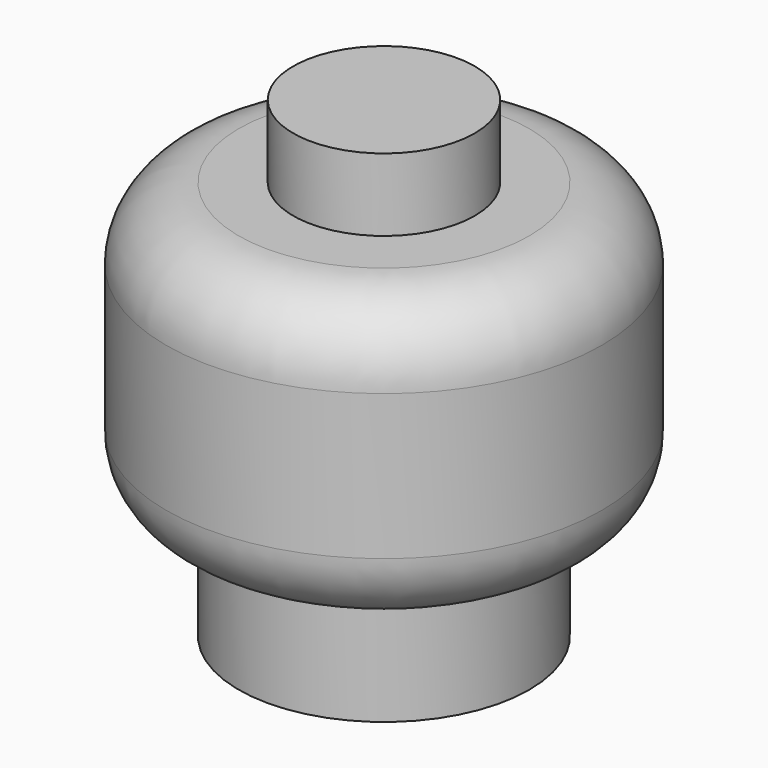
from build123d import *

# Parameters (mm, degrees)
F0_R     = 4
F1_DEPTH = 3
F2_R     = 6
F3_DEPTH = 8
F4_R     = 2.5
F5_DEPTH = 2
F6_R     = 1.99999
F7_R     = 2.5
F8_DEPTH = 2


# Not quite as in the source:
# - a fillet or chamfer is up to 0.001 mm smaller than in the source, because OpenCascade refuses the exact size


with BuildPart() as f1:
    # F0 (on Top) → F1 (new body)
    with BuildSketch(Plane.XY):
        Circle(F0_R)
    extrude(amount=F1_DEPTH)

    # F2 (on face) → F3 (join)
    with BuildSketch(Plane.XY.offset(3)):
        Circle(F2_R)
    extrude(amount=F3_DEPTH)

    # F4 (on face) → F5 (join)
    with BuildSketch(Plane.XY.offset(11)):
        Circle(F4_R)
    extrude(amount=F5_DEPTH)

    # F6 (radius 2 in the source; OpenCascade refuses exactly that, so slightly less here)
    f6_edges = [f1.edges().sort_by_distance(p)[0] for p in [
        (-6, 0, 11),
        (-6, 0, 3),
    ]]
    fillet(f6_edges, radius=F6_R)

    # F7 (on face) → F8 (cut)
    with BuildSketch(Plane(origin=(0, 0, 0), x_dir=(1, 0, 0), z_dir=(0, 0, -1))):
        Circle(F7_R)
    extrude(amount=-F8_DEPTH, mode=Mode.SUBTRACT)


solid = f1.part
